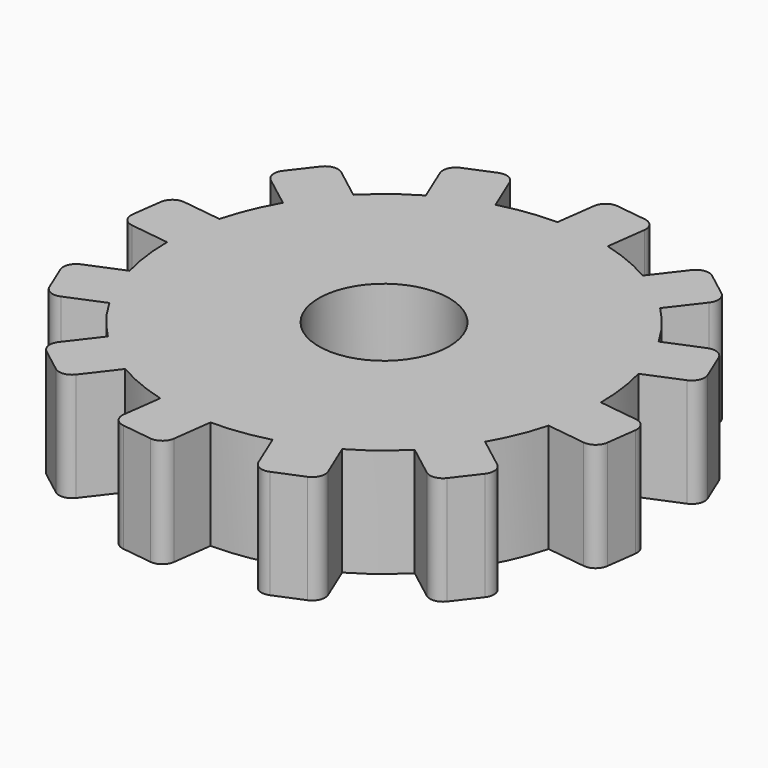
from build123d import *

# Parameters (mm, degrees)
F0_R     = 1.905
F1_DEPTH = 3.175
F2_COUNT = 12


# Not quite as in the source:
# - a length typed as a fraction of an inch, garbled in the dataset ("3 / 203.2 mm" for 3/8 in), is restored


with BuildPart() as f1:
    # F0 (on Top) → F1 (new body)
    with BuildSketch(Plane.XY):
        with BuildLine():
            ThreePointArc((0, 6.3373), (-4.4811478044, -4.4811478044), (6.3373, 0))
            ThreePointArc((6.3373, 0), (5.0277181234, 3.8579038041), (1.6402139345, 6.1213617389))
            ThreePointArc((1.6402139345, 6.1213617389), (0.827183638, 6.28308352), (0, 6.3373))
        make_face()
        Circle(F0_R, mode=Mode.SUBTRACT)
        with BuildLine():
            ThreePointArc((0, 6.3373), (0.827183638, 6.28308352), (1.6402139345, 6.1213617389))
            Line((1.6402139345, 6.1213617389), (1.7907858552, 7.2650690248))
            ThreePointArc((1.7907858552, 7.2650690248), (1.7153129857, 7.5467376085), (1.4627758423, 7.6925399962))
            Line((1.4627758423, 7.6925399962), (0.5780428921, 7.8090172988))
            ThreePointArc((0.5780428921, 7.8090172988), (0.2963743084, 7.7335444293), (0.1505719207, 7.4810072858))
            Line((0.1505719207, 7.4810072858), (0, 6.3373))
        make_face()
    extrude(amount=F1_DEPTH)

    # F2: F1 ×12 about axis
    f2_axis = Axis((0, 0, 0), (0, 0, -1))


with BuildPart() as f1_1:
    add(f1.part)
    for i in range(1, F2_COUNT):
        add(f1.part.rotate(f2_axis, i * 360 / F2_COUNT))


solid = f1_1.part
